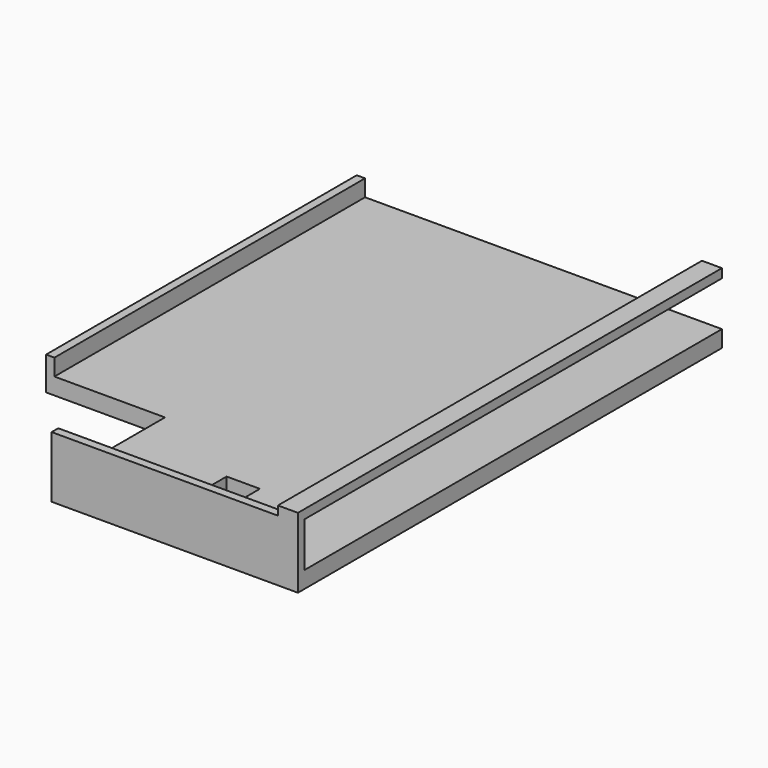
from build123d import *

# Parameters (mm, degrees)
F0_W     = 6.35
F0_H     = 13.716
F1_DEPTH = 3.175
F0_W_2   = 1.5875
F0_H_2   = 73.952875
F2_DEPTH = 6.35
F0_W_3   = 46.9108536
F0_H_3   = 1.5875
F3_DEPTH = 11.684
F6_DEPTH = 3.81


# Not quite as in the source:
# - a feature names something its author has since deleted; it is built from what else it names


with BuildPart() as f1:
    # F0 (on Top) → F1 (new body)
    with BuildSketch(Plane.XY):
        Polygon((33.9837268, -49.6764375), (33.9837268, 49.6764375), (-33.9837268, 49.6764375), (-33.9837268, -24.2764375), (-12.9271268, -24.2764375), (-12.9271268, -49.6764375), align=None)
        with Locations((9.2978732, -40.2784375)):
            Rectangle(F0_W, F0_H, mode=Mode.SUBTRACT)
    extrude(amount=F1_DEPTH)

    # F0 (on Top) → F2 (join)
    with BuildSketch(Plane.XY):
        with Locations((-34.7774768, 12.7)):
            Rectangle(F0_W_2, F0_H_2)
    extrude(amount=F2_DEPTH)

    # F0 (on Top) → F3 (join)
    with BuildSketch(Plane.XY):
        with Locations((10.5283, -50.4701875)):
            Rectangle(F0_W_3, F0_H_3)
    extrude(amount=F3_DEPTH)

    # F5 (on face) → F6 (join)
    with BuildSketch(Plane.YZ.offset(33.9837268)):
        Polygon((-51.2639375, 13.3985), (-51.2639375, 11.684), (-49.6764375, 11.684), (49.6764375, 11.684), (49.6764375, 13.3985), align=None)
    extrude(amount=-F6_DEPTH)


solid = f1.part
